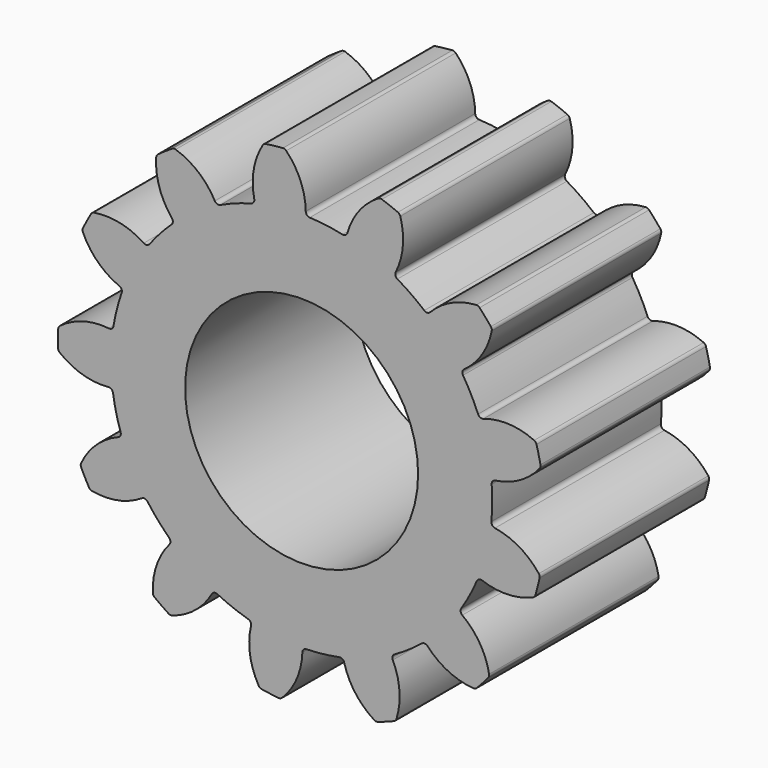
from build123d import *

# Parameters (mm, degrees)
F1_DEPTH = 2
F2_R     = 1.1
F3_DEPTH = 2.001


# Not quite as in the source:
# - a feature names something its author has since deleted; it is built from what else it names


with BuildPart() as f1:
    # F0 (on Front) → F1 (new body)
    with BuildSketch(Plane.XZ):
        with BuildLine():
            ThreePointArc((0.039122928, 1.8376830625), (-0.0105540318, 2.0770952736), (-0.1451690317, 2.2812148684))
            ThreePointArc((-0.1451690317, 2.2812148684), (-0.159702791, 2.2907302121), (-0.1768997755, 2.2931869678))
            ThreePointArc((-0.1768997755, 2.2931869678), (-0.257518295, 2.2855380828), (-0.337817577, 2.2750558861))
            ThreePointArc((-0.337817577, 2.2750558861), (-0.3540367176, 2.2688340373), (-0.366088722, 2.2563231974))
            ThreePointArc((-0.366088722, 2.2563231974), (-0.45190776, 2.0273666515), (-0.4470649859, 1.7829028409))
            ThreePointArc((-0.4470649859, 1.7829028409), (-0.4520346154, 1.7537914646), (-0.475624931, 1.7360244598))
            ThreePointArc((-0.475624931, 1.7360244598), (-0.6237394012, 1.688475395), (-0.7671953061, 1.6283154984))
            ThreePointArc((-0.7671953061, 1.6283154984), (-1.0096932785, 1.4901407595), (-1.2279157548, 1.316139392))
            ThreePointArc((-1.2279157548, 1.316139392), (-1.3369674527, 1.2052045596), (-1.4360336502, 1.0852683334))
            ThreePointArc((-1.4360336502, 1.0852683334), (-1.5865419381, 0.8502262514), (-1.6989058772, 0.5947426506))
            ThreePointArc((-1.6989058772, 0.5947426506), (-1.743912373, 0.4458358839), (-1.775893991, 0.2935992722))
            ThreePointArc((-1.775893991, 0.2935992722), (-1.7999329596, 0.0155351554), (-1.7806971371, -0.2629024645))
            ThreePointArc((-1.7806971371, -0.2629024645), (-1.751347985, -0.4156684199), (-1.7089184204, -0.565329844))
            ThreePointArc((-1.7089184204, -0.565329844), (-1.6009810315, -0.8227148575), (-1.4545521427, -1.0603197934))
            ThreePointArc((-1.4545521427, -1.0603197934), (-1.3575708798, -1.181948098), (-1.2504502343, -1.2947487059))
            ThreePointArc((-1.2504502343, -1.2947487059), (-1.0352636431, -1.4724908113), (-0.7951867816, -1.6148306358))
            ThreePointArc((-0.7951867816, -1.6148306358), (-0.6527906465, -1.6774577109), (-0.5055189691, -1.7275562427))
            ThreePointArc((-0.5055189691, -1.7275562427), (-0.2323798303, -1.7849368657), (0.0463462881, -1.7994032404))
            ThreePointArc((0.0463462881, -1.7994032404), (0.201536057, -1.7886819778), (0.3552205997, -1.7646014637))
            ThreePointArc((0.3552205997, -1.7646014637), (0.6237394012, -1.688475395), (0.8772619817, -1.5717542478))
            ThreePointArc((0.8772619817, -1.5717542478), (1.0096932785, -1.4901407595), (1.13458341, -1.397397755))
            ThreePointArc((1.13458341, -1.397397755), (1.3369674527, -1.2052045596), (1.5072075275, -0.9840352987))
            ThreePointArc((1.5072075275, -0.9840352987), (1.5865419381, -0.8502262514), (1.6540268343, -0.7100670611))
            ThreePointArc((1.6540268343, -0.7100670611), (1.743912373, -0.4458358839), (1.7918699925, -0.1708857215))
            ThreePointArc((1.7918699925, -0.1708857215), (1.7999329596, -0.0155351554), (1.7945526441, 0.1399314392))
            ThreePointArc((1.7945526441, 0.1399314392), (1.751347985, 0.4156684199), (1.6660366367, 0.681411715))
            ThreePointArc((1.6660366367, 0.681411715), (1.6009810315, 0.8227148575), (1.5239680698, 0.9578733332))
            ThreePointArc((1.5239680698, 0.9578733332), (1.3575708798, 1.181948098), (1.1585343652, 1.3776059395))
            ThreePointArc((1.1585343652, 1.3776059395), (1.0352636431, 1.4724908113), (0.9042607765, 1.5563779901))
            ThreePointArc((0.9042607765, 1.5563779901), (0.6527906465, 1.6774577109), (0.3856258326, 1.7582072452))
            ThreePointArc((0.3856258326, 1.7582072452), (0.2323798303, 1.7849368657), (0.0773982368, 1.7983352059))
            ThreePointArc((0.0773982368, 1.7983352059), (0.0504458492, 1.8104074157), (0.039122928, 1.8376830625))
        make_face()
        with BuildLine():
            ThreePointArc((-1.2279157548, 1.316139392), (-1.0096932785, 1.4901407595), (-0.7671953061, 1.6283154984))
            ThreePointArc((-0.7671953061, 1.6283154984), (-0.7966706958, 1.6264795102), (-0.8193722697, 1.6453688721))
            ThreePointArc((-0.8193722697, 1.6453688721), (-0.9746194353, 1.8342718227), (-1.1886742036, 1.9524520381))
            ThreePointArc((-1.1886742036, 1.9524520381), (-1.2059652091, 1.9541232819), (-1.222334094, 1.9483067938))
            ThreePointArc((-1.222334094, 1.9483067938), (-1.2901636337, 1.9040687483), (-1.3563937971, 1.8574702871))
            ThreePointArc((-1.3563937971, 1.8574702871), (-1.3678636956, 1.8444237031), (-1.3727211383, 1.8277450588))
            ThreePointArc((-1.3727211383, 1.8277450588), (-1.3423087103, 1.5851320101), (-1.2244126493, 1.3709206053))
            ThreePointArc((-1.2244126493, 1.3709206053), (-1.2152843065, 1.3428342597), (-1.2279157548, 1.316139392))
        make_face()
        with BuildLine():
            ThreePointArc((-1.7806971371, -0.2629024645), (-1.7999329596, 0.0155351554), (-1.775893991, 0.2935992722))
            ThreePointArc((-1.775893991, 0.2935992722), (-1.7911269321, 0.2682985419), (-1.819568536, 0.2603458935))
            ThreePointArc((-1.819568536, 0.2603458935), (-2.0632230584, 0.2398890878), (-2.2820804367, 0.1308594811))
            ThreePointArc((-2.2820804367, 0.1308594811), (-2.293278254, 0.1175786373), (-2.2977899646, 0.1008031673))
            ThreePointArc((-2.2977899646, 0.1008031673), (-2.2999143372, 0.0198504764), (-2.2991875764, -0.0611268226))
            ThreePointArc((-2.2991875764, -0.0611268226), (-2.2949660933, -0.0779776684), (-2.2839991801, -0.0914498153))
            ThreePointArc((-2.2839991801, -0.0914498153), (-2.0670563272, -0.2042407978), (-1.8237912011, -0.2289001891))
            ThreePointArc((-1.8237912011, -0.2289001891), (-1.7954911021, -0.2373425731), (-1.7806971371, -0.2629024645))
        make_face()
        with BuildLine():
            ThreePointArc((-0.7951867816, -1.6148306358), (-1.0352636431, -1.4724908113), (-1.2504502343, -1.2947487059))
            ThreePointArc((-1.2504502343, -1.2947487059), (-1.2382814383, -1.3216576237), (-1.2478932095, -1.349582224))
            ThreePointArc((-1.2478932095, -1.349582224), (-1.369469133, -1.5617267549), (-1.404064687, -1.8037787221))
            ThreePointArc((-1.404064687, -1.8037787221), (-1.399495852, -1.8205387242), (-1.3882528546, -1.8337813424))
            ThreePointArc((-1.3882528546, -1.8337813424), (-1.3228368773, -1.8815160366), (-1.2557810195, -1.9269182731))
            ThreePointArc((-1.2557810195, -1.9269182731), (-1.2395149695, -1.933016432), (-1.2221976933, -1.9316438911))
            ThreePointArc((-1.2221976933, -1.9316438911), (-1.0061349477, -1.8171760042), (-0.8476503242, -1.6309808612))
            ThreePointArc((-0.8476503242, -1.6309808612), (-0.8246260898, -1.612486157), (-0.7951867816, -1.6148306358))
        make_face()
        with BuildLine():
            ThreePointArc((0.0073975122, -1.8380845787), (0.0191895417, -1.8110084362), (0.0463462881, -1.7994032404))
            ThreePointArc((0.0463462881, -1.7994032404), (-0.2323798303, -1.7849368657), (-0.5055189691, -1.7275562427))
            ThreePointArc((-0.5055189691, -1.7275562427), (-0.4822388378, -1.7457277846), (-0.4777724297, -1.774920603))
            ThreePointArc((-0.4777724297, -1.774920603), (-0.4868340843, -2.019264405), (-0.4049797681, -2.2496681335))
            ThreePointArc((-0.4049797681, -2.2496681335), (-0.3931455043, -2.2623851349), (-0.377036173, -2.2688860095))
            ThreePointArc((-0.377036173, -2.2688860095), (-0.2969297831, -2.2807526617), (-0.2164552985, -2.2897919346))
            ThreePointArc((-0.2164552985, -2.2897919346), (-0.1992184707, -2.2876323759), (-0.1845226357, -2.2783693117))
            ThreePointArc((-0.1845226357, -2.2783693117), (-0.0464044552, -2.076603667), (0.0073975122, -1.8380845787))
        make_face()
        with BuildLine():
            ThreePointArc((0.8607506676, -1.6241052705), (0.8586090804, -1.5946505077), (0.8772619817, -1.5717542478))
            ThreePointArc((0.8772619817, -1.5717542478), (0.6237394012, -1.688475395), (0.3552205997, -1.7646014637))
            ThreePointArc((0.3552205997, -1.7646014637), (0.3842788689, -1.7698727484), (0.401800256, -1.793646062))
            ThreePointArc((0.401800256, -1.793646062), (0.5073287861, -2.0142129148), (0.6868811351, -2.180185687))
            ThreePointArc((0.6868811351, -2.180185687), (0.7032697406, -2.1859463759), (0.7205549521, -2.1842162349))
            ThreePointArc((0.7205549521, -2.1842162349), (0.7970003459, -2.157496338), (0.8724577228, -2.1281018589))
            ThreePointArc((0.8724577228, -2.1281018589), (0.8867165788, -2.1181793113), (0.8954243339, -2.1031477803))
            ThreePointArc((0.8954243339, -2.1031477803), (0.9239567387, -1.8603064554), (0.8607506676, -1.6241052705))
        make_face()
        with BuildLine():
            ThreePointArc((1.5169162183, -1.0380630175), (1.5013316261, -1.0129773655), (1.5072075275, -0.9840352987))
            ThreePointArc((1.5072075275, -0.9840352987), (1.3369674527, -1.2052045596), (1.13458341, -1.397397755))
            ThreePointArc((1.13458341, -1.397397755), (1.1627629177, -1.3885611948), (1.1893253453, -1.401468824))
            ThreePointArc((1.1893253453, -1.401468824), (1.3852687455, -1.5477295196), (1.6213858481, -1.6112489736))
            ThreePointArc((1.6213858481, -1.6112489736), (1.6385743632, -1.6087336456), (1.6530756213, -1.5991688436))
            ThreePointArc((1.6530756213, -1.5991688436), (1.7083473006, -1.5399836039), (1.7615011941, -1.4788892938))
            ThreePointArc((1.7615011941, -1.4788892938), (1.7695155463, -1.4634768934), (1.7702403797, -1.4461204381))
            ThreePointArc((1.7702403797, -1.4461204381), (1.6826505787, -1.2178354541), (1.5169162183, -1.0380630175))
        make_face()
        with BuildLine():
            ThreePointArc((1.8255745442, -0.2142130372), (1.8001171894, -0.1992433165), (1.7918699925, -0.1708857215))
            ThreePointArc((1.7918699925, -0.1708857215), (1.743912373, -0.4458358839), (1.6540268343, -0.7100670611))
            ThreePointArc((1.6540268343, -0.7100670611), (1.6748719949, -0.6891470055), (1.7043903309, -0.6882319679))
            ThreePointArc((1.7043903309, -0.6882319679), (1.9458603297, -0.7266799437), (2.1844506031, -0.6731945381))
            ThreePointArc((2.1844506031, -0.6731945381), (2.1985013461, -0.6629794245), (2.2068965874, -0.6477711422))
            ThreePointArc((2.2068965874, -0.6477711422), (2.2283324766, -0.569679185), (2.2470059702, -0.4908810139))
            ThreePointArc((2.2470059702, -0.4908810139), (2.2469398271, -0.473509556), (2.2395156882, -0.4578043312))
            ThreePointArc((2.2395156882, -0.4578043312), (2.0558694492, -0.2963730267), (1.8255745442, -0.2142130372))
        make_face()
        with BuildLine():
            ThreePointArc((1.7160157425, 0.6587105685), (1.6865175983, 0.6601349751), (1.6660366367, 0.681411715))
            ThreePointArc((1.6660366367, 0.681411715), (1.751347985, 0.4156684199), (1.7945526441, 0.1399314392))
            ThreePointArc((1.7945526441, 0.1399314392), (1.8032880825, 0.1681424577), (1.8290000318, 0.1826705379))
            ThreePointArc((1.8290000318, 0.1826705379), (2.0606787625, 0.2608432499), (2.2470840504, 0.4190806532))
            ThreePointArc((2.2470840504, 0.4190806532), (2.2547781655, 0.434655393), (2.2551441412, 0.4520231213))
            ThreePointArc((2.2551441412, 0.4520231213), (2.2378335365, 0.5311318698), (2.2177487579, 0.6095821904))
            ThreePointArc((2.2177487579, 0.6095821904), (2.209617272, 0.6249331143), (2.1957449416, 0.6353892309))
            ThreePointArc((2.1957449416, 0.6353892309), (1.9581134048, 0.6929848894), (1.7160157425, 0.6587105685))
        make_face()
        with BuildLine():
            ThreePointArc((1.2133384145, 1.3807315211), (1.1865571502, 1.3682842994), (1.1585343652, 1.3776059395))
            ThreePointArc((1.1585343652, 1.3776059395), (1.3575708798, 1.181948098), (1.5239680698, 0.9578733332))
            ThreePointArc((1.5239680698, 0.9578733332), (1.5185926024, 0.9869125101), (1.5346078672, 1.0117254249))
            ThreePointArc((1.5346078672, 1.0117254249), (1.7034205247, 1.1886103985), (1.794937622, 1.4153495174))
            ThreePointArc((1.794937622, 1.4153495174), (1.7945124802, 1.4327158981), (1.7867653498, 1.4482643352))
            ThreePointArc((1.7867653498, 1.4482643352), (1.7346739019, 1.5102670141), (1.6804320319, 1.5703974612))
            ThreePointArc((1.6804320319, 1.5703974612), (1.6660980287, 1.5802111393), (1.6489554905, 1.5830227774))
            ThreePointArc((1.6489554905, 1.5830227774), (1.4117771772, 1.5235883187), (1.2133384145, 1.3807315211))
        make_face()
        with BuildLine():
            ThreePointArc((0.432699878, 1.786443522), (0.4147707585, 1.7629761804), (0.3856258326, 1.7582072452))
            ThreePointArc((0.3856258326, 1.7582072452), (0.6527906465, 1.6774577109), (0.9042607765, 1.5563779901))
            ThreePointArc((0.9042607765, 1.5563779901), (0.886005858, 1.5795928001), (0.8886555343, 1.6090062097))
            ThreePointArc((0.8886555343, 1.6090062097), (0.9559291731, 1.844081229), (0.9315926158, 2.0873788639))
            ThreePointArc((0.9315926158, 2.0873788639), (0.9231456119, 2.1025584571), (0.9090601496, 2.1127256434))
            ThreePointArc((0.9090601496, 2.1127256434), (0.8341213816, 2.1434181862), (0.7581485788, 2.171453599))
            ThreePointArc((0.7581485788, 2.171453599), (0.7408958057, 2.173481836), (0.7244102086, 2.1680048831))
            ThreePointArc((0.7244102086, 2.1680048831), (0.5420198121, 2.0051560255), (0.432699878, 1.786443522))
        make_face()
        with BuildLine():
            ThreePointArc((-1.6989058772, 0.5947426506), (-1.5865419381, 0.8502262514), (-1.4360336502, 1.0852683334))
            ThreePointArc((-1.4360336502, 1.0852683334), (-1.4612795853, 1.0699447501), (-1.4901591549, 1.076120502))
            ThreePointArc((-1.4901591549, 1.076120502), (-1.7154112715, 1.1712388026), (-1.9598684406, 1.1764059755))
            ThreePointArc((-1.9598684406, 1.1764059755), (-1.9759555312, 1.1698502574), (-1.9877464022, 1.1570930129))
            ThreePointArc((-1.9877464022, 1.1570930129), (-2.027248032, 1.0864002101), (-2.0642365445, 1.0143606302))
            ThreePointArc((-2.0642365445, 1.0143606302), (-2.0683295854, 0.9974781262), (-2.0648796848, 0.9804525539))
            ThreePointArc((-2.0648796848, 0.9804525539), (-1.9252029116, 0.7797627281), (-1.7212621305, 0.6448769804))
            ThreePointArc((-1.7212621305, 0.6448769804), (-1.7001270088, 0.6242499088), (-1.6989058772, 0.5947426506))
        make_face()
        with BuildLine():
            ThreePointArc((-1.4545521427, -1.0603197934), (-1.6009810315, -0.8227148575), (-1.7089184204, -0.565329844))
            ThreePointArc((-1.7089184204, -0.565329844), (-1.7106486842, -0.5948116288), (-1.7321366938, -0.6150708217))
            ThreePointArc((-1.7321366938, -0.6150708217), (-1.9383753071, -0.7464163261), (-2.0814953069, -0.9446653433))
            ThreePointArc((-2.0814953069, -0.9446653433), (-2.0852385658, -0.9616288317), (-2.0814375375, -0.9785794691))
            ThreePointArc((-2.0814375375, -0.9785794691), (-2.0456979847, -1.0512467623), (-2.0074224428, -1.122610857))
            ThreePointArc((-2.0074224428, -1.122610857), (-1.9958535266, -1.135569719), (-1.9798819884, -1.1424021339))
            ThreePointArc((-1.9798819884, -1.1424021339), (-1.7353720489, -1.1414552182), (-1.5085116865, -1.0502390838))
            ThreePointArc((-1.5085116865, -1.0502390838), (-1.4795298219, -1.0445627318), (-1.4545521427, -1.0603197934))
        make_face()
    extrude(amount=F1_DEPTH)

    # F2 (on face) → F3 (cut, through all)
    with BuildSketch(Plane.XZ.offset(2)):
        Circle(F2_R)
    extrude(amount=-F3_DEPTH, mode=Mode.SUBTRACT)


solid = f1.part
